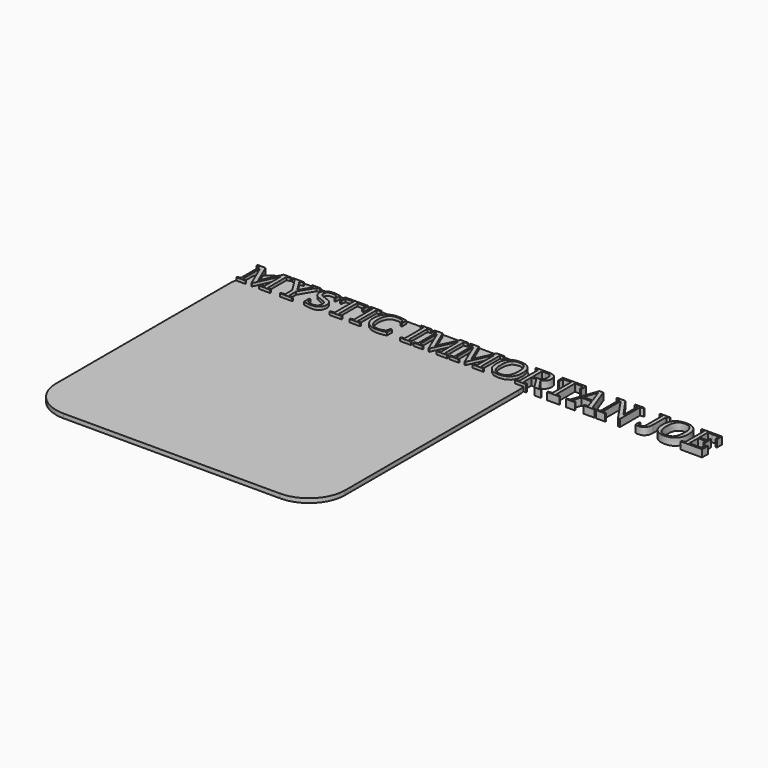
from build123d import *

# Parameters (mm, degrees)
F1_DEPTH     = 1.4986
F2_TEXT_SIZE = 14.2708192647
F3_DEPTH     = 2.54


# Not quite as in the source:
# - Text() gives the source's letters only with a copy of the font that has no kerning and outlines rounded to 1/6400 em; it was checked with that copy


with BuildPart() as f1:
    # F0 (on Top) → F1 (new body)
    with BuildSketch(Plane.XY):
        with BuildLine():
            Line((88.9, 0), (12.7, 0))
            ThreePointArc((12.7, 0), (3.7197438789, -3.7197438789), (0, -12.7))
            Line((0, -12.7), (0, -88.9))
            ThreePointArc((0, -88.9), (3.7197438789, -97.8802561211), (12.7, -101.6))
            Line((12.7, -101.6), (88.9, -101.6))
            ThreePointArc((88.9, -101.6), (97.8802561211, -97.8802561211), (101.6, -88.9))
            Line((101.6, -88.9), (101.6, -12.7))
            ThreePointArc((101.6, -12.7), (97.8802561211, -3.7197438789), (88.9, 0))
        make_face()
    extrude(amount=F1_DEPTH)


with BuildPart() as f3:
    # F2 (on Top) → F3 (new body)
    with BuildSketch(Plane.XY):
        with Locations((0, -10.2749898706)):
            Text('MYSTIC IMMORTAN JOE', F2_TEXT_SIZE, font='Tinos', text_align=(TextAlign.LEFT, TextAlign.BOTTOM))
    extrude(amount=F3_DEPTH)


solid = Compound([f1.part, f3.part])
